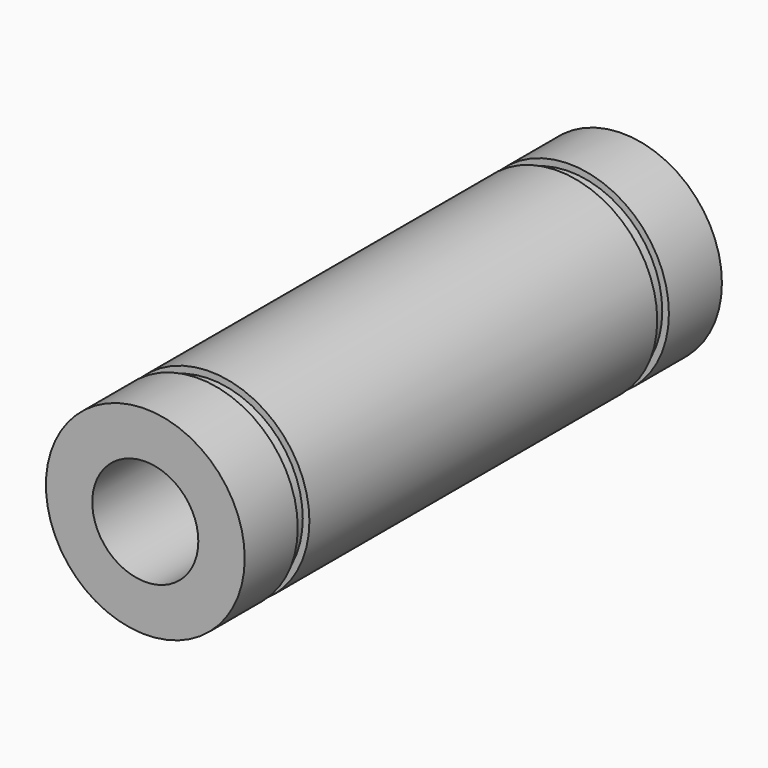
from build123d import *

# Parameters (mm, degrees)
F0_R     = 7.5
F0_R_2   = 4
F1_DEPTH = 5
F2_R     = 7
F2_R_2   = 4
F3_DEPTH = 1.1
F4_R     = 7.5
F4_R_2   = 7
F4_R_3   = 4
F5_DEPTH = 32.8
F6_R     = 7
F6_R_2   = 4
F7_DEPTH = 1.1
F8_R     = 7.5
F8_R_2   = 7
F8_R_3   = 4
F9_DEPTH = 5


# Not quite as in the source:
# - a feature names something its author has since deleted; it is built from what else it names


with BuildPart() as f1:
    # F0 (on Front) → F1 (new body)
    with BuildSketch(Plane.XZ):
        Circle(F0_R)
        Circle(F0_R_2, mode=Mode.SUBTRACT)
    extrude(amount=F1_DEPTH)

    # F2 (on face) → F3 (join)
    with BuildSketch(Plane.XZ.offset(5)):
        Circle(F2_R)
        Circle(F2_R_2, mode=Mode.SUBTRACT)
    extrude(amount=F3_DEPTH)

    # F4 (on face) → F5 (join)
    with BuildSketch(Plane.XZ.offset(6.1)):
        Circle(F4_R)
        Circle(F4_R_2, mode=Mode.SUBTRACT)
        Circle(F4_R_2)
        Circle(F4_R_3, mode=Mode.SUBTRACT)
    extrude(amount=F5_DEPTH)

    # F6 (on face) → F7 (join)
    with BuildSketch(Plane.XZ.offset(38.9)):
        Circle(F6_R)
        Circle(F6_R_2, mode=Mode.SUBTRACT)
    extrude(amount=F7_DEPTH)

    # F8 (on face) → F9 (join)
    with BuildSketch(Plane.XZ.offset(40)):
        Circle(F8_R)
        Circle(F8_R_2, mode=Mode.SUBTRACT)
        Circle(F8_R_2)
        Circle(F8_R_3, mode=Mode.SUBTRACT)
    extrude(amount=F9_DEPTH)


solid = f1.part
